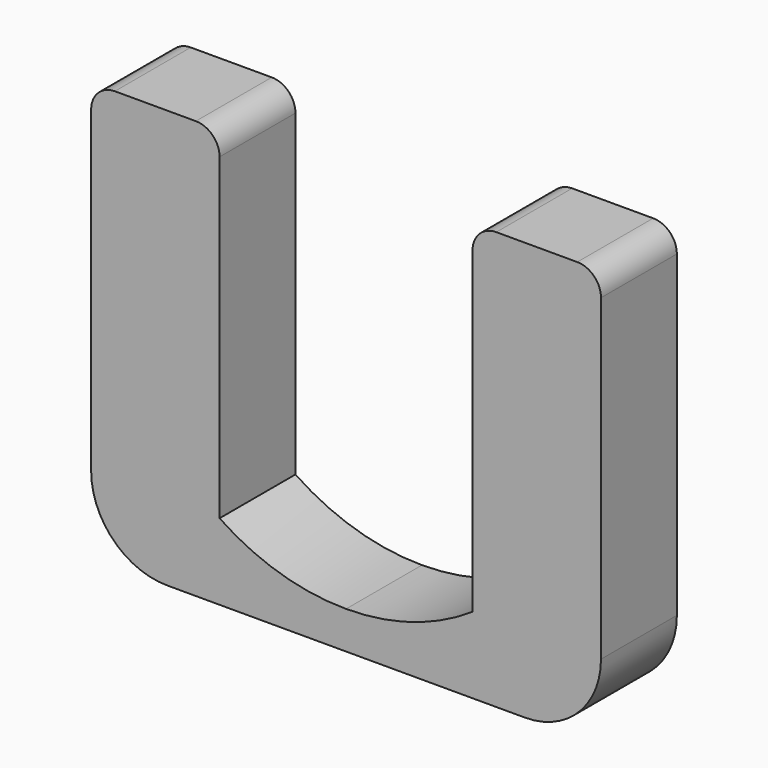
from build123d import *

# Parameters (mm, degrees)
F1_DEPTH = 25.4


# Not quite as in the source:
# - the program builds the solid bodies; features that only make, move or delete a surface that nothing else refers to are left out


with BuildPart() as f1:
    # F0 (on Front) → F1 (new body)
    with BuildSketch(Plane.XZ):
        with BuildLine():
            ThreePointArc((0, -25.9232582643), (-17.7094384525, -23.2773241348), (-33.8721087757, -15.5706214843))
            Line((-33.8721087757, -15.5706214843), (-68.2603194002, -15.5706214843))
            ThreePointArc((-68.2603194002, -15.5706214843), (-62.2686711741, -30.0120658628), (-47.8133782744, -35.9702259302))
            Line((-47.8133782744, -35.9702259302), (0, -35.9702259302))
            Line((0, -35.9702259302), (47.8133782744, -35.9702259302))
            ThreePointArc((47.8133782744, -35.9702259302), (62.2686711741, -30.0120658628), (68.2603194002, -15.5706214843))
            Line((68.2603194002, -15.5706214843), (33.8721087757, -15.5706214843))
            ThreePointArc((33.8721087757, -15.5706214843), (17.7094384525, -23.2773241348), (0, -25.9232582643))
        make_face()
        with BuildLine():
            Line((-68.2603194002, -15.5706214843), (-33.8721087757, -15.5706214843))
            Line((-33.8721087757, -15.5706214843), (-33.8721087757, 69.6263722184))
            ThreePointArc((-33.8721087757, 69.6263722184), (-35.7319807152, 74.1165002789), (-40.2221087757, 75.9763722184))
            Line((-40.2221087757, 75.9763722184), (-61.9103194002, 75.9763722184))
            ThreePointArc((-61.9103194002, 75.9763722184), (-66.4004474607, 74.1165002789), (-68.2603194002, 69.6263722184))
            Line((-68.2603194002, 69.6263722184), (-68.2603194002, -15.5706214843))
        make_face()
        with BuildLine():
            Line((33.8721087757, 69.6263722184), (33.8721087757, -15.5706214843))
            Line((33.8721087757, -15.5706214843), (68.2603194002, -15.5706214843))
            Line((68.2603194002, -15.5706214843), (68.2603194002, 69.6263722184))
            ThreePointArc((68.2603194002, 69.6263722184), (66.4004474607, 74.1165002789), (61.9103194002, 75.9763722184))
            Line((61.9103194002, 75.9763722184), (40.2221087757, 75.9763722184))
            ThreePointArc((40.2221087757, 75.9763722184), (35.7319807152, 74.1165002789), (33.8721087757, 69.6263722184))
        make_face()
    extrude(amount=F1_DEPTH)


solid = f1.part
